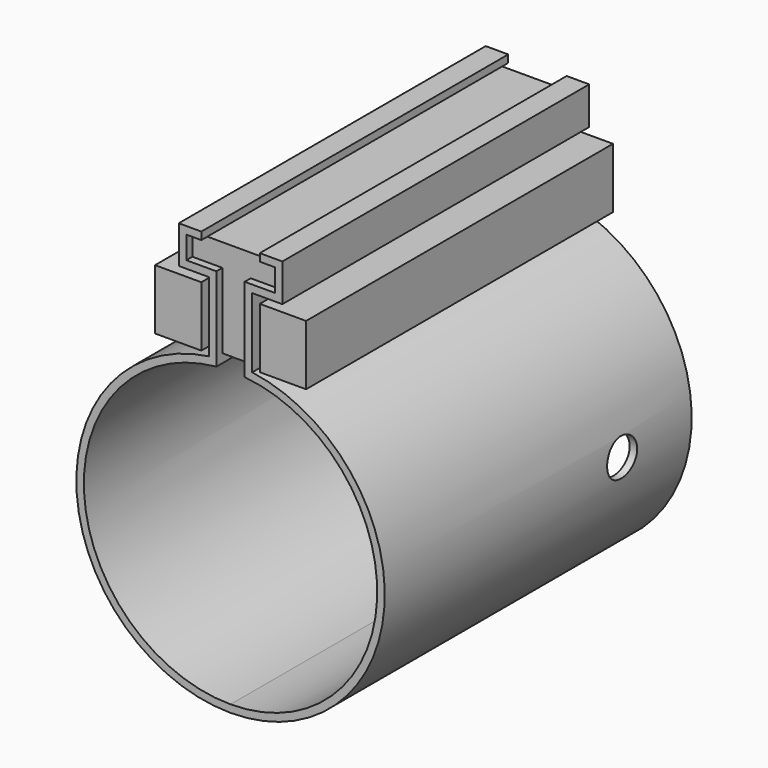
from build123d import *

# Parameters (mm, degrees)
F0_W      = 1
F0_H      = 7
F1_DEPTH  = 25.5
F2_W      = 1
F2_H      = 7
F3_DEPTH  = 3
F4_W      = 1
F4_H      = 7
F5_DEPTH  = 3
F7_DEPTH  = 1
F9_DEPTH  = 1
F13_D     = 5
F13_DEPTH = 6
F13_TIP   = 1.5021515476


# Not quite as in the source:
# - a pattern or mirror of a feature is missing from the dataset's text; its kind, count and spacing are read off the source's solid


with BuildPart() as f1:
    # F0 (on Front) → F1 (new body, symmetric)
    with BuildSketch(Plane.XZ):
        with BuildLine():
            ThreePointArc((1.8823727184, 19.4089328132), (19.4772198973, -0.9422871488), (0, -19.5))
            Line((0, -19.5), (0, -20.5))
            ThreePointArc((0, -20.5), (20.4490247642, -1.444778942), (2.8823727184, 20.2963525667))
            Line((2.8823727184, 20.2963525667), (2.8823727184, 21.2562642992))
            Line((2.8823727184, 21.2562642992), (2.8823727184, 28.2562642992))
            Line((2.8823727184, 28.2562642992), (2.8823727184, 29.5688871337))
            Line((2.8823727184, 29.5688871337), (6.8823727184, 29.5688871337))
            Line((6.8823727184, 29.5688871337), (6.8823727184, 34.5688871337))
            Line((6.8823727184, 34.5688871337), (3.8823727184, 34.5688871337))
            Line((3.8823727184, 34.5688871337), (3.8823727184, 33.5702374578))
            Line((3.8823727184, 33.5702374578), (3.8823727184, 33.5688871337))
            Line((3.8823727184, 33.5688871337), (5.8823727184, 33.5688871337))
            Line((5.8823727184, 33.5688871337), (5.8823727184, 30.5688871337))
            Line((5.8823727184, 30.5688871337), (1.8823727184, 30.5688871337))
            Line((1.8823727184, 30.5688871337), (1.8823727184, 20.578497021))
            Line((1.8823727184, 20.578497021), (1.8823727184, 19.4089328132))
        make_face()
        Polygon((0, 20.561426878), (1.8823727184, 20.578497021), (1.8823727184, 30.5688871337), (5.8823727184, 30.5688871337), (5.8823727184, 33.5688871337), (3.8823727184, 33.5688871337), (3.8823727184, 33.5702374578), (0, 33.5702374578), align=None)
        with Locations((3.3823727184, 24.7562642992)):
            Rectangle(F0_W, F0_H)
        Polygon((3.8823727184, 28.2562642992), (3.8823727184, 21.2562642992), (3.8823727184, 20.6377897412), (10.0385518745, 20.6377897412), (10.0385518745, 28.6377897412), (3.8823727184, 28.6377897412), align=None)
    extrude(amount=F1_DEPTH, both=True)

    # F2 (on face) → F3 (cut)
    with BuildSketch(Plane.XZ.offset(25.5)):
        with Locations((3.3823727184, 24.7562642992)):
            Rectangle(F2_W, F2_H)
    extrude(amount=-F3_DEPTH, mode=Mode.SUBTRACT)

    # F4 (on face) → F5 (cut)
    with BuildSketch(Plane(origin=(0, 25.5, 0), x_dir=(-1, 0, 0), z_dir=(0, 1, 0))):
        with Locations((-3.3823727184, 24.7562642992)):
            Rectangle(F4_W, F4_H)
    extrude(amount=-F5_DEPTH, mode=Mode.SUBTRACT)

    # F6 (on face) → F7 (cut)
    with BuildSketch(Plane.XZ.offset(25.5)):
        Polygon((0, 20.561426878), (1.8823727184, 20.578497021), (1.8823727184, 30.5688871337), (5.8823727184, 30.5688871337), (5.8823727184, 33.5688871337), (3.8823727184, 33.5688871337), (3.8823727184, 33.5702374578), (0, 33.5702374578), align=None)
    extrude(amount=-F7_DEPTH, mode=Mode.SUBTRACT)

    # F8 (on face) → F9 (cut)
    with BuildSketch(Plane(origin=(0, 25.5, 0), x_dir=(-1, 0, 0), z_dir=(0, 1, 0))):
        Polygon((-1.8823727184, 30.5688871337), (-1.8823727184, 20.578497021), (0, 20.561426878), (0, 33.5702374578), (-3.8823727184, 33.5702374578), (-3.8823727184, 33.5688871337), (-5.8823727184, 33.5688871337), (-5.8823727184, 30.5688871337), align=None)
    extrude(amount=-F9_DEPTH, mode=Mode.SUBTRACT)

    # F10: F1 across plane


with BuildPart() as f1_1:
    add(f1.part)
    add(f1.part.mirror(Plane.YZ))

    # F13
    with Locations(Plane(origin=(-20.5, 0, 0), x_dir=(0, 1, 0), z_dir=(-1, 0, 0))):
        with Locations((13.9512377791, 0)):
            f13 = Hole(F13_D / 2, depth=F13_DEPTH)
            with Locations((0, 0, -(F13_DEPTH + F13_TIP / 2))):  # 118° drill point
                Cone(0, F13_D / 2, F13_TIP, mode=Mode.SUBTRACT)

    # F13_copies: F13 across plane
    add(f13.mirror(Plane(origin=(-1.9e-05, 0, 0), x_dir=(0, 0, 1), z_dir=(1, 0, 0))), mode=Mode.SUBTRACT)


solid = f1_1.part
